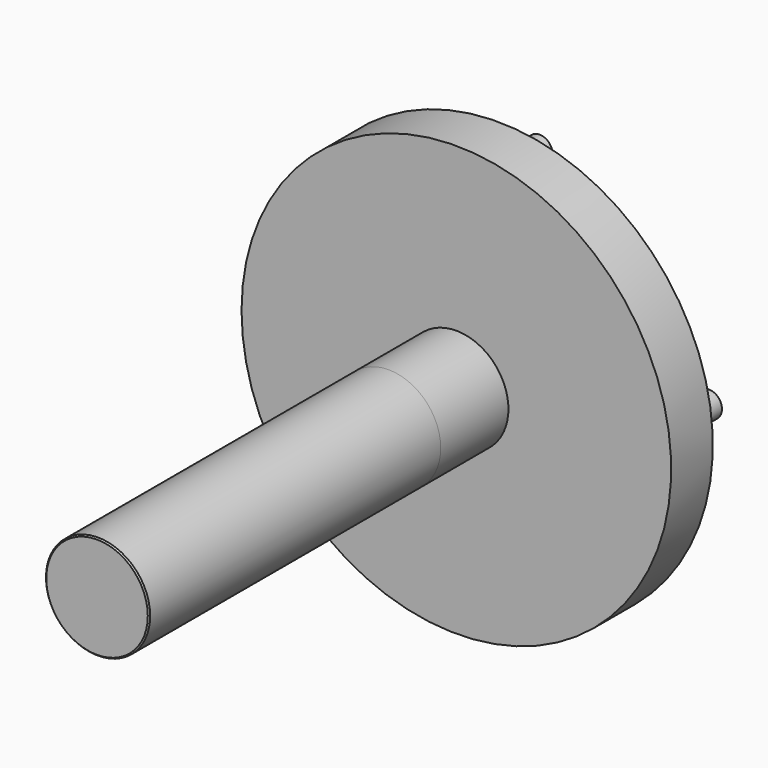
from build123d import *

# Parameters (mm, degrees)
F0_R     = 4
F1_DEPTH = 28
F2_SIZE  = 0.1
F3_R     = 4
F4_DEPTH = 6.5
F5_R     = 16.5
F6_DEPTH = 4
F7_R     = 1
F8_DEPTH = 4


with BuildPart() as f1:
    # F0 (on Front) → F1 (new body)
    with BuildSketch(Plane.XZ):
        Circle(F0_R)
    extrude(amount=-F1_DEPTH)

    # F2
    f2_edges = [f1.edges().sort_by_distance(p)[0] for p in [
        (-4, 0, 0),
    ]]
    chamfer(f2_edges, length=F2_SIZE)

    # F3 (on face) → F4 (join)
    with BuildSketch(Plane(origin=(0, 28, 0), x_dir=(-1, 0, 0), z_dir=(0, 1, 0))):
        Circle(F3_R)
    extrude(amount=F4_DEPTH)

    # F5 (on face) → F6 (join)
    with BuildSketch(Plane(origin=(0, 34.5, 0), x_dir=(-1, 0, 0), z_dir=(0, 1, 0))):
        Circle(F5_R)
    extrude(amount=F6_DEPTH)

    # F7 (on face) → F8 (join)
    with BuildSketch(Plane(origin=(0, 38.5, 0), x_dir=(-1, 0, 0), z_dir=(0, 1, 0))):
        with Locations((0, 13)):
            Circle(F7_R)
        with Locations((-13, 0)):
            Circle(F7_R)
        with Locations((0, -13)):
            Circle(F7_R)
        with Locations((13, 0)):
            Circle(F7_R)
    extrude(amount=F8_DEPTH)


solid = f1.part
